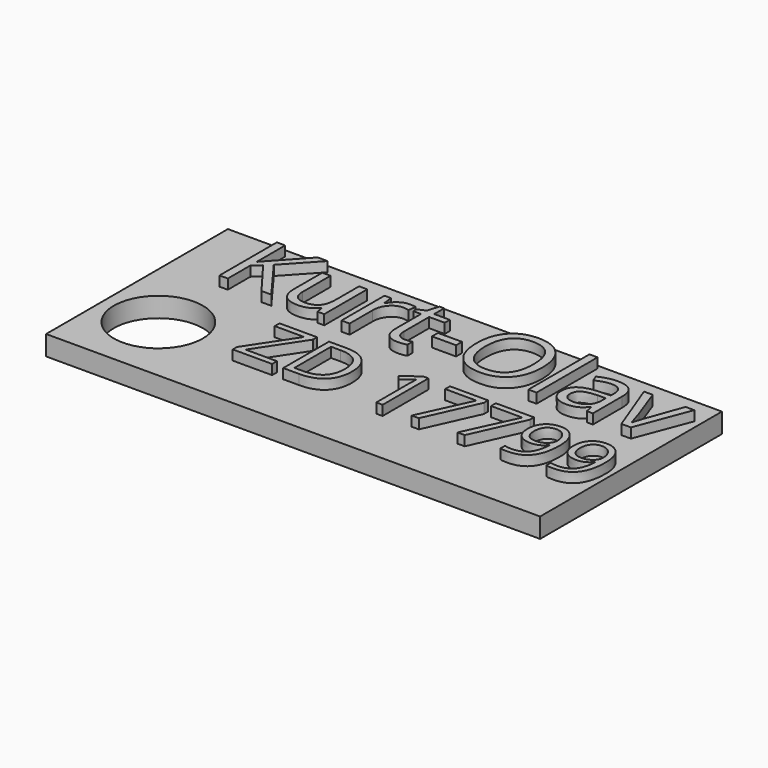
from build123d import *

# Parameters (mm, degrees)
F0_W           = 50
F0_H           = 23
F1_DEPTH       = 2
F2_TEXT_SIZE   = 10.160372276
F3_DEPTH       = 1
F4_TEXT_SIZE   = 8.1174925917
F5_DEPTH       = 1
F7_D           = 3
F7_CBORE_D     = 9
F7_CBORE_DEPTH = 2


# Not quite as in the source:
# - Text() gives the source's letters only with a copy of the font that has no kerning and outlines rounded to 1/6400 em; it was checked with that copy


with BuildPart() as f1:
    # F0 (on Top) → F1 (new body)
    with BuildSketch(Plane.XY):
        Rectangle(F0_W, F0_H)
    extrude(amount=F1_DEPTH)

    # F2 (on face) → F3 (join)
    with BuildSketch(Plane.XY.offset(2)):
        with Locations((-20.3565368635, 3.3878813308)):
            Text('Kurt-Olav', F2_TEXT_SIZE, font='Open Sans', text_align=(TextAlign.LEFT, TextAlign.BOTTOM))
    extrude(amount=F3_DEPTH)

    # F4 (on face) → F5 (join)
    with BuildSketch(Plane.XY.offset(2)):
        with Locations((-10.9566871064, -5.844594666)):
            Text('ZD 17799', F4_TEXT_SIZE, font='Open Sans', text_align=(TextAlign.LEFT, TextAlign.BOTTOM))
    extrude(amount=F5_DEPTH)

    # F7 (through all)
    with Locations(Plane.XY.offset(2)):
        with Locations((-19.3445719779, -4.3632304296)):
            CounterBoreHole(F7_D / 2, F7_CBORE_D / 2, F7_CBORE_DEPTH)


solid = f1.part
